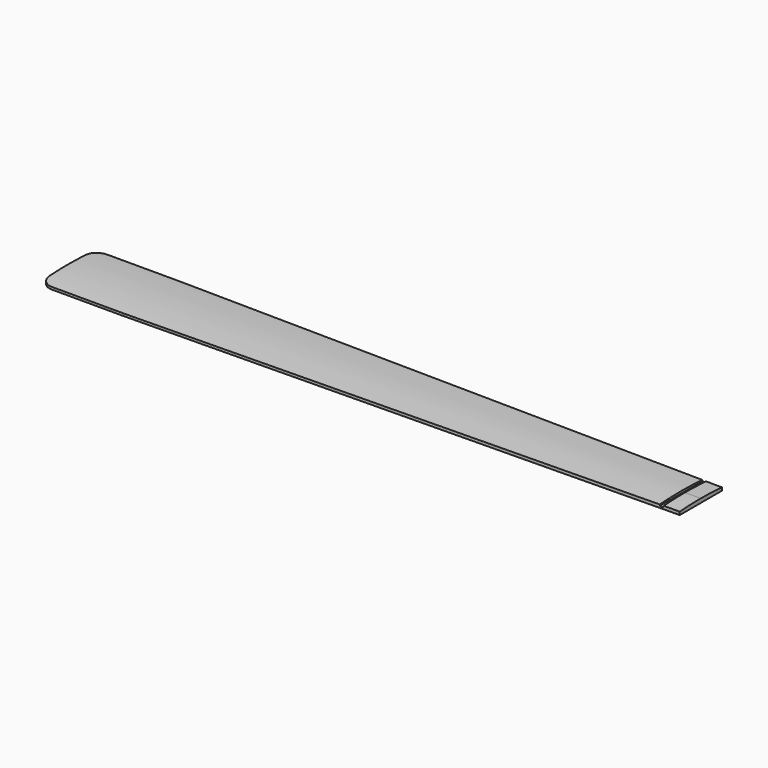
from build123d import *

# Parameters (mm, degrees)
F2_DEPTH      = 3.81
F3_W          = 3.048
F3_H          = 50.8
F4_DEPTH      = 2.38125
F6_DEPTH      = 330.597875
F6_DEPTH_BACK = 208.8139096404
F7_W          = 63.5
F7_H          = 127
F8_DEPTH      = 3.8110001


# Not quite as in the source:
# - ends of sketch curves that miss each other by under 0.0002 mm in the source are joined


with BuildPart() as f2:
    # F1 (on Top) → F2 (new body)
    with BuildSketch(Plane.XY):
        with BuildLine():
            Line((-321.071875, -27.78125), (-264.9117892, -27.78125))
            ThreePointArc((-264.9117892, -27.78125), (-263.9219083354, -27.7773922086), (-262.9320876087, -27.7658190689))
            Line((-262.9320876087, -27.7658190689), (171.053125, -21.0000088))
            ThreePointArc((171.053125, -21.0000088), (193.158824833, -26.9518731046), (208.8129096404, -43.6562539958))
            Line((208.8129096404, -43.6562539958), (208.8129096404, 43.6562539958))
            ThreePointArc((208.8129096404, 43.6562539958), (193.158824833, 26.9518731046), (171.053124933, 21.0000041509))
            Line((171.053124933, 21.0000041509), (-262.9320878, 27.7658068))
            ThreePointArc((-262.9320878, 27.7658068), (-263.9219083354, 27.7773922086), (-264.9117892, 27.78125))
            Line((-264.9117892, 27.78125), (-321.071875, 27.78125))
            ThreePointArc((-321.071875, 27.78125), (-327.8070670908, 24.9914420908), (-330.596875, 18.25625))
            Line((-330.596875, 18.25625), (-330.596875, -18.25625))
            ThreePointArc((-330.596875, -18.25625), (-327.8070670908, -24.9914420908), (-321.071875, -27.78125))
        make_face()
    extrude(amount=F2_DEPTH)

    # F3 (on face) → F4 (cut)
    with BuildSketch(Plane.XY.offset(3.81)):
        with Locations((159.877125, 0)):
            Rectangle(F3_W, F3_H)
    extrude(amount=-F4_DEPTH, mode=Mode.SUBTRACT)

    # F5 (on Right) → F6 (cut, two sides)
    with BuildSketch(Plane.YZ) as f6_sk:
        with BuildLine():
            Line((38.1, 15.875), (0, 15.875))
            Line((0, 15.875), (-38.1, 15.875))
            Line((-38.1, 15.875), (-38.1, 0.7843748547))
            ThreePointArc((-38.1, 0.7843748547), (-19.0874637432, 2.5767566153), (0, 3.175))
            ThreePointArc((0, 3.175), (19.0874637432, 2.5767566153), (38.1, 0.7843748547))
            Line((38.1, 0.7843748547), (38.1, 15.875))
        make_face()
    extrude(amount=-F6_DEPTH, mode=Mode.SUBTRACT)
    extrude(f6_sk.sketch, amount=F6_DEPTH_BACK, mode=Mode.SUBTRACT)

    # F7 (on Top) → F8 (cut, through all)
    with BuildSketch(Plane.XY):
        with Locations((205.851125, 0)):
            Rectangle(F7_W, F7_H)
    extrude(amount=F8_DEPTH, mode=Mode.SUBTRACT)


solid = f2.part
